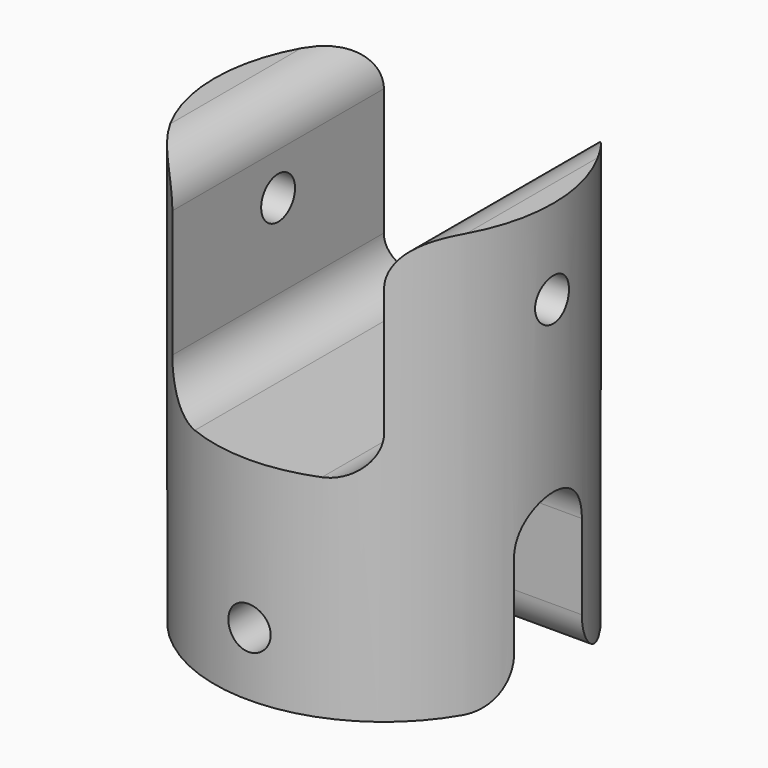
from build123d import *

# Parameters (mm, degrees)
F0_R      = 8
F1_DEPTH  = 10
F3_DEPTH  = 10
F5_D      = 2
F5_DEPTH  = 8.001
F6_D      = 2
F7_R      = 2
F9_DEPTH  = 8
F10_R     = 1.9999
F11_R     = 1
F12_DEPTH = 8


# Not quite as in the source:
# - a fillet or chamfer is up to 0.001 mm smaller than in the source, because OpenCascade refuses the exact size
# - a feature names something its author has since deleted; it is built from what else it names


with BuildPart() as f1:
    # F0 (on Top) → F1 (new body, symmetric)
    with BuildSketch(Plane.XY):
        Circle(F0_R)
    extrude(amount=F1_DEPTH, both=True)

    # F2 (on face) → F3 (cut)
    with BuildSketch(Plane.XY.offset(10)):
        with BuildLine():
            ThreePointArc((5, 6.2449979984), (0, 8), (-5, 6.2449979984))
            Line((-5, 6.2449979984), (-5, -6.2449979984))
            ThreePointArc((-5, -6.2449979984), (0, -8), (5, -6.2449979984))
            Line((5, -6.2449979984), (5, 6.2449979984))
        make_face()
    extrude(amount=-F3_DEPTH, mode=Mode.SUBTRACT)

    # F5 (through all, one way)
    with BuildSketch(Plane.YZ):
        with Locations((0, 6)):
            Circle(F5_D / 2)
    extrude(amount=-F5_DEPTH, mode=Mode.SUBTRACT)

    # F6 (through all)
    with Locations(Plane(origin=(0, 0, 0), x_dir=(0, 1, 0), z_dir=(-1, 0, 0))):
        with Locations((0, -6)):
            Hole(F6_D / 2)

    # F7
    f7_edges = [f1.edges().sort_by_distance(p)[0] for p in [
        (5, 0, 10),
        (-5, 0, 10),
    ]]
    fillet(f7_edges, radius=F7_R)

    # F8 (on face) → F9 (cut)
    with BuildSketch(Plane(origin=(0, 0, -10), x_dir=(1, 0, 0), z_dir=(0, 0, -1))):
        with BuildLine():
            Line((7.7459666924, 2), (-7.7459666924, 2))
            ThreePointArc((-7.7459666924, 2), (-8, 0), (-7.7459666924, -2))
            Line((-7.7459666924, -2), (7.7459666924, -2))
            ThreePointArc((7.7459666924, -2), (7.9362375701, -1.0080343399), (8, 0))
            ThreePointArc((8, 0), (7.9362375701, 1.0080343399), (7.7459666924, 2))
        make_face()
    extrude(amount=-F9_DEPTH, mode=Mode.SUBTRACT)

    # F10 (radius 2 in the source; OpenCascade refuses exactly that, so slightly less here)
    f10_edges = [f1.edges().sort_by_distance(p)[0] for p in [
        (0, 2, -10),
        (0, -2, -10),
        (0, -2, -2),
        (0, 2, -2),
        (-5, 0, 0),
        (5, 0, 0),
    ]]
    fillet(f10_edges, radius=F10_R)

    # F11 (on Front) → F12 (cut, symmetric)
    with BuildSketch(Plane.XZ):
        with Locations((0, -7)):
            Circle(F11_R)
    extrude(amount=F12_DEPTH, both=True, mode=Mode.SUBTRACT)


solid = f1.part
